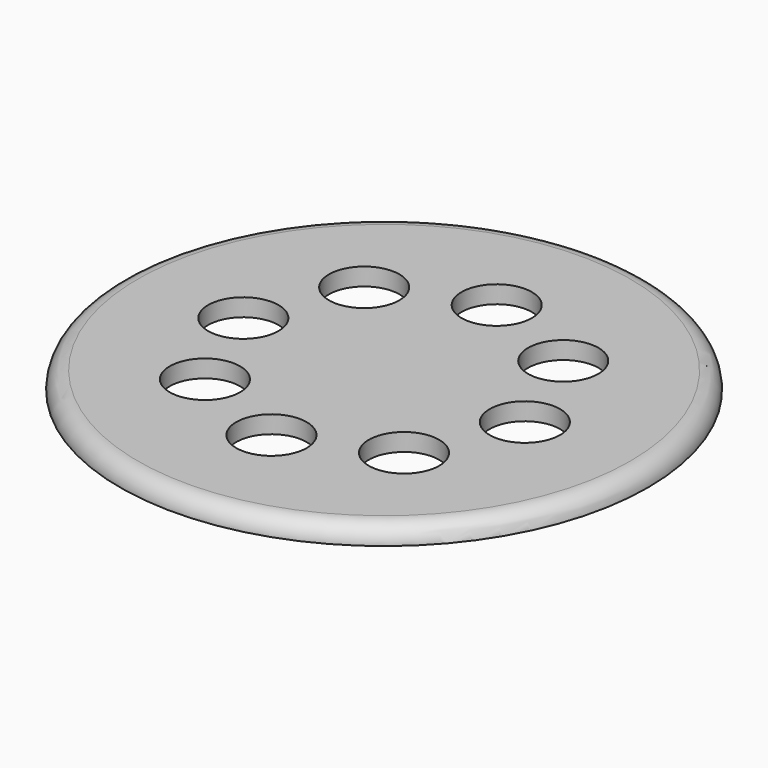
from build123d import *

# Parameters (mm, degrees)
F0_R     = 75
F0_R_2   = 10
F1_DEPTH = 5
F2_R     = 4.99999


# Not quite as in the source:
# - a fillet or chamfer is up to 0.001 mm smaller than in the source, because OpenCascade refuses the exact size
# - the program builds the solid bodies; features that only make, move or delete a surface that nothing else refers to are left out


with BuildPart() as f1:
    # F0 (on Top) → F1 (new body)
    with BuildSketch(Plane.XY):
        Circle(F0_R)
        with Locations((-28.2842712475, -28.2842712475)):
            Circle(F0_R_2, mode=Mode.SUBTRACT)
        with Locations((0, -40)):
            Circle(F0_R_2, mode=Mode.SUBTRACT)
        with Locations((28.2842712475, -28.2842712475)):
            Circle(F0_R_2, mode=Mode.SUBTRACT)
        with Locations((-40, 0)):
            Circle(F0_R_2, mode=Mode.SUBTRACT)
        with Locations((-28.2842712475, 28.2842712475)):
            Circle(F0_R_2, mode=Mode.SUBTRACT)
        with Locations((28.2842712475, 28.2842712475)):
            Circle(F0_R_2, mode=Mode.SUBTRACT)
        with Locations((40, 0)):
            Circle(F0_R_2, mode=Mode.SUBTRACT)
        with Locations((0, 40)):
            Circle(F0_R_2, mode=Mode.SUBTRACT)
    extrude(amount=F1_DEPTH)

    # F2 (radius 5 in the source; OpenCascade refuses exactly that, so slightly less here)
    f2_edges = [f1.edges().sort_by_distance(p)[0] for p in [
        (-75, 0, 5),
    ]]
    fillet(f2_edges, radius=F2_R)


solid = f1.part
